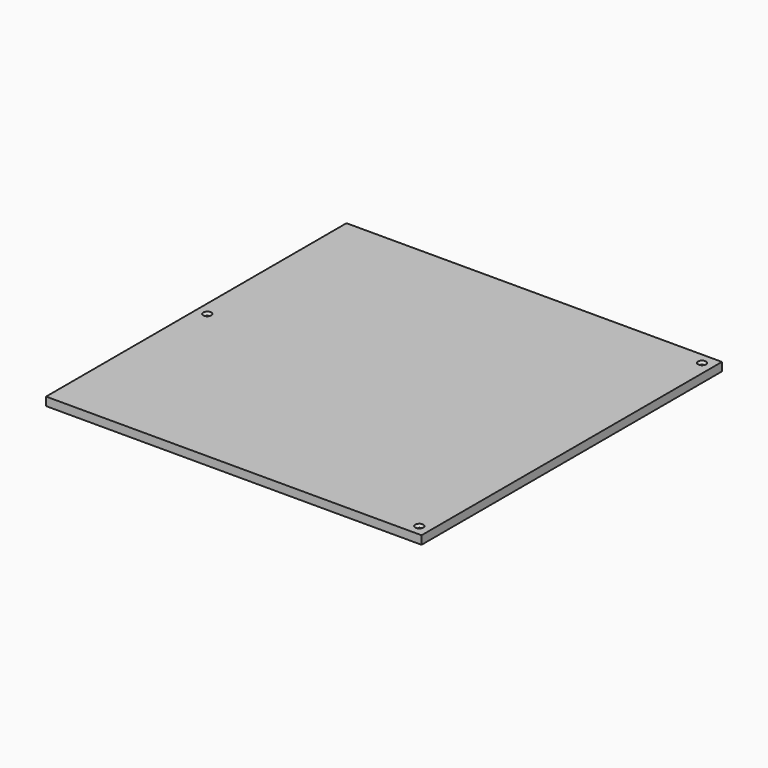
from build123d import *

# Parameters (mm, degrees)
F0_W           = 425
F0_H           = 425
F1_DEPTH       = 9.525
F2_R           = 200
F3_DEPTH       = 1
F5_D           = 4.318
F5_CSINK_D     = 9.1186
F5_CSINK_ANGLE = 82


# Not quite as in the source:
# - a length typed as a fraction of an inch, garbled in the dataset ("3 / 203.2 mm" for 3/8 in), is restored


with BuildPart() as f1:
    # F0 (on Top) → F1 (new body)
    with BuildSketch(Plane.XY):
        Rectangle(F0_W, F0_H)
    extrude(amount=-F1_DEPTH)

    # F5 (through all)
    with Locations(Plane.XY):
        with Locations((200, -200), (200, 200), (-200, 0)):
            CounterSinkHole(F5_D / 2, F5_CSINK_D / 2, counter_sink_angle=F5_CSINK_ANGLE)


with BuildPart() as f3:
    # F2 (on face) → F3 (new body)
    with BuildSketch(Plane(origin=(0, 0, -9.525), x_dir=(1, 0, 0), z_dir=(0, 0, -1))):
        Circle(F2_R)
    extrude(amount=F3_DEPTH)


solid = Compound([f1.part, f3.part])
